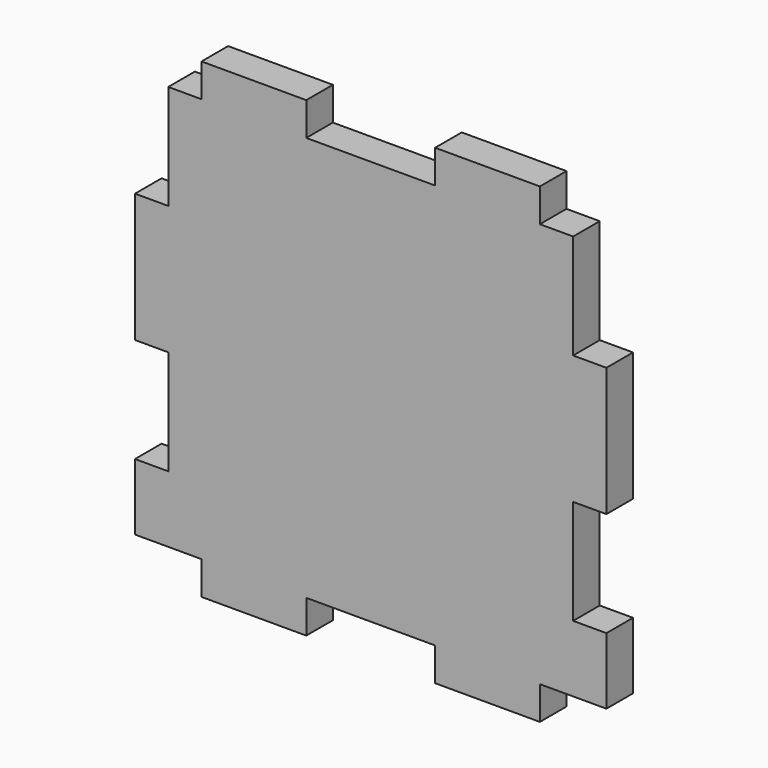
from build123d import *

# Parameters (mm, degrees)
F0_W     = 1.5875
F0_H     = 12.3
F1_DEPTH = 3.175


# Not quite as in the source:
# - a length typed as a fraction of an inch, garbled in the dataset ("3 / 203.2 mm" for 3/8 in), is restored
# - a feature names something its author has since deleted; it is built from what else it names


with BuildPart() as f1:
    # F0 (on Front) → F1 (new body)
    with BuildSketch(Plane.XZ):
        with Locations((21.70625, 0)):
            Rectangle(F0_W, F0_H)
        with Locations((-21.70625, 0)):
            Rectangle(F0_W, F0_H)
        Polygon((-22.5, -16.15), (-22.5, -22.5), (-16.15, -22.5), (-16.15, -25.675), (-6.15, -25.675), (-6.15, -22.5), (6.15, -22.5), (6.15, -25.675), (16.15, -25.675), (16.15, -22.5), (22.5, -22.5), (22.5, -16.15), (19.325, -16.15), (19.325, -6.15), (20.9125, -6.15), (20.9125, 6.15), (19.325, 6.15), (19.325, 16.15), (16.15, 16.15), (16.15, 19.325), (6.15, 19.325), (6.15, 16.15), (-6.15, 16.15), (-6.15, 19.325), (-16.15, 19.325), (-16.15, 16.15), (-19.325, 16.15), (-19.325, 6.15), (-20.9125, 6.15), (-20.9125, -6.15), (-19.325, -6.15), (-19.325, -16.15), align=None)
    extrude(amount=F1_DEPTH)


solid = f1.part
